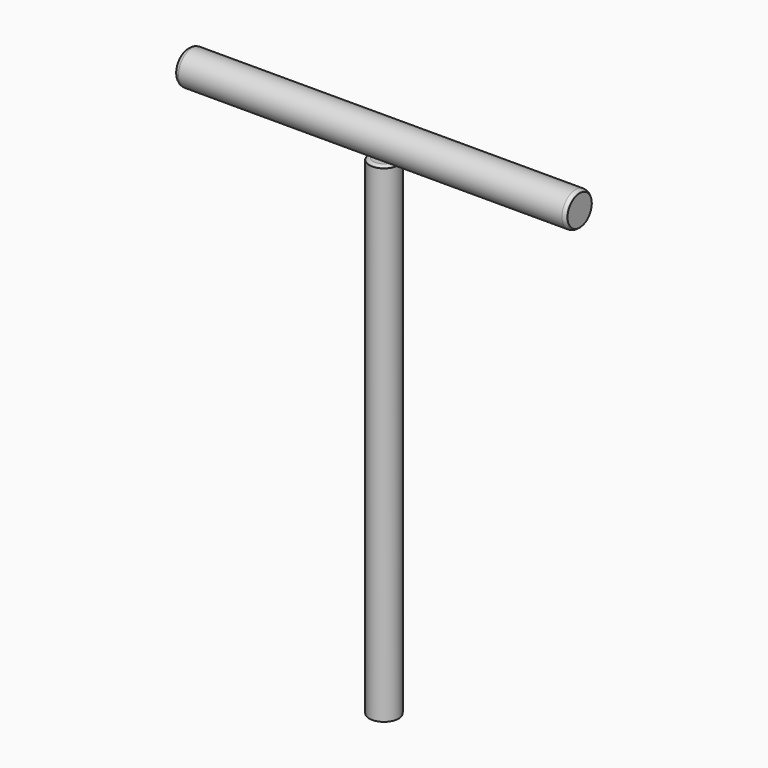
from build123d import *

# Parameters (mm, degrees)
F0_R           = 15
F1_DEPTH       = 500
F2_R           = 17.5
F3_DEPTH       = 200
F4_T2_ANGLE    = 180
F4_T4_ANGLE    = 180
F4_S1_C1_SIZE  = 2
F4_S1_C2_SIZE  = 2
F5_F1_R        = 5
F5_F2_R        = 5
F5_S1_T2_ANGLE = 180
F5_S1_T4_ANGLE = 180


# Not quite as in the source:
# - a fillet or chamfer that OpenCascade refuses, or shapes differently, is made with other operations: its cross-section is extruded or revolved along the edge and cut away or added


with BuildPart() as f1:
    # F0 (on Top) → F1 (new body)
    with BuildSketch(Plane.XY):
        Circle(F0_R)
    extrude(amount=-F1_DEPTH)

    # F2 (on Right) → F3 (join, symmetric)
    with BuildSketch(Plane.YZ):
        with Locations((0, 17.5)):
            Circle(F2_R)
    extrude(amount=F3_DEPTH, both=True)

    # F4: chamfer of 2 on 3 edges, made by hand

    # F4_s1 → F4_t2 (revolve, cut)
    with BuildSketch(Plane.XZ):
        Polygon((15, -2), (13, 0), (15, 0), align=None)
    revolve(axis=Axis((0, 0, 0), (0, 0, 1)), revolution_arc=F4_T2_ANGLE, mode=Mode.SUBTRACT)

    # F4_s3 → F4_t4 (revolve, cut)
    with BuildSketch(Plane.XZ):
        Polygon((-15, -2), (-13, 0), (-15, 0), align=None)
    revolve(axis=Axis((0, 0, 0), (0, 0, 1)), revolution_arc=F4_T4_ANGLE, mode=Mode.SUBTRACT)

    # F4#s1: chamfer of 2 on 3 edges, made by hand

    # F4_s1_c1
    f4_s1_c1_edges = [f1.edges().sort_by_distance(p)[0] for p in [
        (200, -17.5, 17.5),
    ]]
    chamfer(f4_s1_c1_edges, length=F4_S1_C1_SIZE)

    # F4_s1_c2
    f4_s1_c2_edges = [f1.edges().sort_by_distance(p)[0] for p in [
        (-200, -17.5, 17.5),
    ]]
    chamfer(f4_s1_c2_edges, length=F4_S1_C2_SIZE)

    # F5: fillet of radius 5 on 6 edges, made by hand

    # F5_f1
    f5_f1_edges = [f1.edges().sort_by_distance(p)[0] for p in [
        (-198, -17.5, 17.5),
    ]]
    fillet(f5_f1_edges, radius=F5_F1_R)

    # F5_f2
    f5_f2_edges = [f1.edges().sort_by_distance(p)[0] for p in [
        (198, -17.5, 17.5),
    ]]
    fillet(f5_f2_edges, radius=F5_F2_R)

    # F5#s1: fillet of radius 5 on 2 edges, made by hand

    # F5_s1_s1 → F5_s1_t2 (revolve, cut)
    with BuildSketch(Plane.XZ):
        with BuildLine():
            ThreePointArc((-14.4644660941, -1.4644660941), (-12.84234935, -0.3806023374), (-10.9289321881, 0))
            Line((-10.9289321881, 0), (-13, 0))
            Line((-13, 0), (-14.4644660941, -1.4644660941))
        make_face()
    revolve(axis=Axis((0, 0, 0), (0, 0, 1)), revolution_arc=F5_S1_T2_ANGLE, mode=Mode.SUBTRACT)

    # F5_s1_s3 → F5_s1_t4 (revolve, cut)
    with BuildSketch(Plane.XZ):
        with BuildLine():
            ThreePointArc((14.4644660941, -1.4644660941), (12.84234935, -0.3806023374), (10.9289321881, 0))
            Line((10.9289321881, 0), (13, 0))
            Line((13, 0), (14.4644660941, -1.4644660941))
        make_face()
    revolve(axis=Axis((0, 0, 0), (0, 0, 1)), revolution_arc=F5_S1_T4_ANGLE, mode=Mode.SUBTRACT)


solid = f1.part
